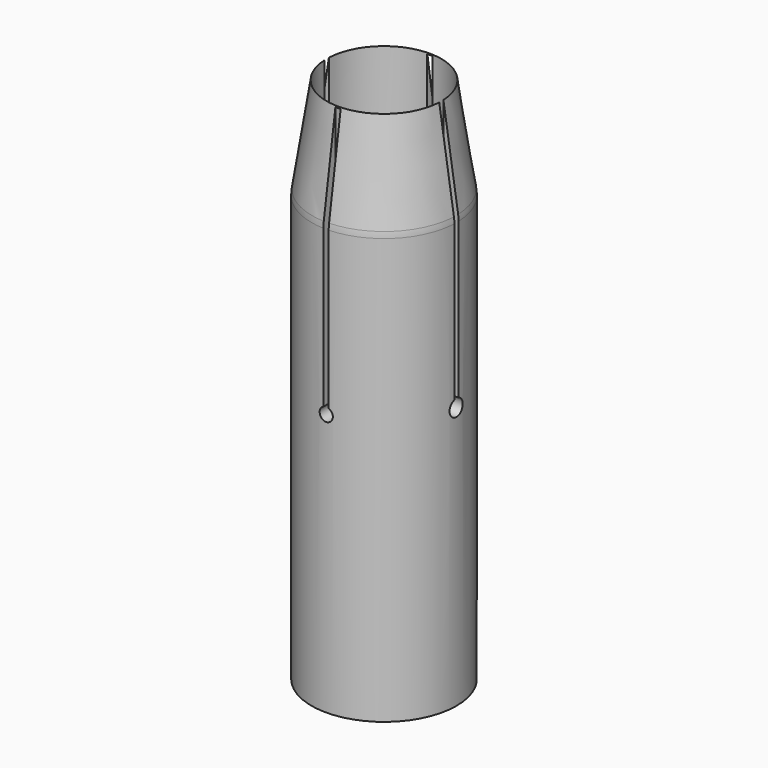
from build123d import *

# Parameters (mm, degrees)
F3_R      = 2.54
F4_SIZE   = 2.54
F5_SIZE   = 3.17499
F6_R      = 7.62
F7_W      = 1.016
F7_H      = 50.8
F8_DEPTH  = 13.9710001
F9_DEPTH  = 25.4
F10_R     = 1.27
F11_DEPTH = 13.9710001
F12_DEPTH = 13.9710001
F13_W     = 1.016
F13_H     = 57.15
F14_DEPTH = 13.9710001
F15_DEPTH = 13.9710001001
F16_R     = 1.5875
F17_DEPTH = 13.9710001
F18_DEPTH = 13.9710001


# Not quite as in the source:
# - a fillet or chamfer is up to 0.001 mm smaller than in the source, because OpenCascade refuses the exact size


with BuildPart() as f2:
    # F0 (on Front) → F2 (revolve)
    with BuildSketch(Plane.XZ):
        Polygon((10.795, 39.9480294436), (10.795, 0), (13.97, 0), (13.97, 82.55), (11.049, 101.6), (11.049, 83.3468958735), (11.684, 69.85), (12.319, 69.85), (12.319, 67.691), (11.684, 67.691), (11.049, 47.371), (7.62, 47.371), (7.62, 39.9480294436), align=None)
    revolve(axis=Axis((0, 0, 18.4564618394), (0, 0, 1)))

    # F3
    f3_edges = [f2.edges().sort_by_distance(p)[0] for p in [
        (-10.795, 0, 0),
    ]]
    fillet(f3_edges, radius=F3_R)

    # F4
    f4_edges = [f2.edges().sort_by_distance(p)[0] for p in [
        (-7.62, 0, 47.371),
    ]]
    chamfer(f4_edges, length=F4_SIZE)

    # F5 (size 3.175 in the source; OpenCascade refuses exactly that, so slightly less here)
    f5_edges = [f2.edges().sort_by_distance(p)[0] for p in [
        (-10.795, 0, 39.948029),
    ]]
    chamfer(f5_edges, length=F5_SIZE)

    # F6
    f6_edges = [f2.edges().sort_by_distance(p)[0] for p in [
        (-13.97, 0, 82.55),
    ]]
    fillet(f6_edges, radius=F6_R)

    # F7 (on Front) → F8 (cut, through all)
    with BuildSketch(Plane.XZ):
        with Locations((0, 75.946)):
            Rectangle(F7_W, F7_H)
    extrude(amount=-F8_DEPTH, mode=Mode.SUBTRACT)

    # F7 (on Front) → F9 (cut)
    with BuildSketch(Plane.XZ):
        with Locations((0, 75.946)):
            Rectangle(F7_W, F7_H)
    extrude(amount=F9_DEPTH, mode=Mode.SUBTRACT)

    # F10 (on Front) → F11 (cut, through all)
    with BuildSketch(Plane.XZ):
        with Locations((0, 50.546)):
            Circle(F10_R)
    extrude(amount=-F11_DEPTH, mode=Mode.SUBTRACT)

    # F10 (on Front) → F12 (cut, through all)
    with BuildSketch(Plane.XZ):
        with Locations((0, 50.546)):
            Circle(F10_R)
    extrude(amount=F12_DEPTH, mode=Mode.SUBTRACT)

    # F13 (on Right) → F14 (cut, through all)
    with BuildSketch(Plane.YZ):
        with Locations((0, 79.13624)):
            Rectangle(F13_W, F13_H)
    extrude(amount=-F14_DEPTH, mode=Mode.SUBTRACT)

    # F13 (on Right) → F15 (cut, through all)
    with BuildSketch(Plane.YZ):
        with Locations((0, 79.13624)):
            Rectangle(F13_W, F13_H)
    extrude(amount=F15_DEPTH, mode=Mode.SUBTRACT)

    # F16 (on Right) → F17 (cut, through all)
    with BuildSketch(Plane.YZ):
        with Locations((0, 50.56124)):
            Circle(F16_R)
    extrude(amount=-F17_DEPTH, mode=Mode.SUBTRACT)

    # F16 (on Right) → F18 (cut, through all)
    with BuildSketch(Plane.YZ):
        with Locations((0, 50.56124)):
            Circle(F16_R)
    extrude(amount=F18_DEPTH, mode=Mode.SUBTRACT)


solid = f2.part
